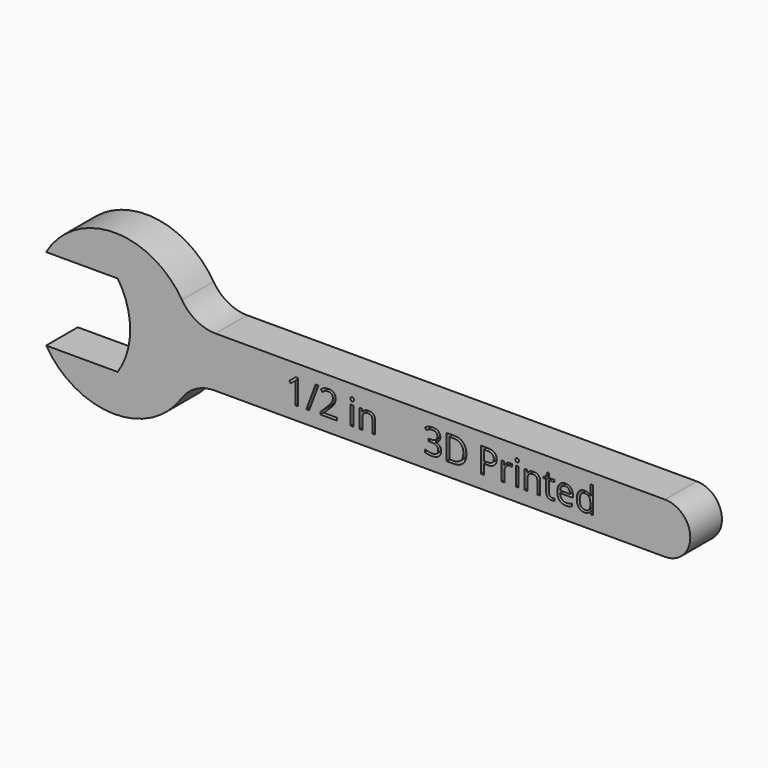
from build123d import *

# Parameters (mm, degrees)
F1_DEPTH     = 6.35
F2_TEXT_SIZE = 5.5941565531
F3_DEPTH     = 2


# Not quite as in the source:
# - Text() gives the source's letters only with a copy of the font that has no kerning and outlines rounded to 1/6400 em; it was checked with that copy


with BuildPart() as f1:
    # F0 (on Front) → F1 (new body)
    with BuildSketch(Plane.XZ):
        with BuildLine():
            Line((53.5489660396, 8.1024769281), (-18.6246478565, 8.1024769281))
            ThreePointArc((-18.6246478565, 8.1024769281), (-21.707286584, 8.900915123), (-24.0147138151, 11.0954411877))
            ThreePointArc((-24.0147138151, 11.0954411877), (-35.014283693, 17.0959234193), (-45.8292585891, 10.7687880083))
            Line((-45.8292585891, 10.7687880083), (-34.3312044384, 10.7687880083))
            ThreePointArc((-34.3312044384, 10.7687880083), (-32.3274172275, 4.1647880083), (-34.3312044384, -2.4392119917))
            Line((-34.3312044384, -2.4392119917), (-45.8206947839, -2.4392119917))
            ThreePointArc((-45.8206947839, -2.4392119917), (-35.0509770881, -8.5655910788), (-24.0725254588, -2.8216429775))
            ThreePointArc((-24.0725254588, -2.8216429775), (-21.7861297168, -0.7496621936), (-18.7930182164, 0))
            Line((-18.7930182164, 0), (53.5489660396, 0))
            Line((53.5489660396, 0), (53.5489660396, 8.1024769281))
        make_face()
        with BuildLine():
            ThreePointArc((53.5489660396, 0), (57.6002045036, 4.051238464), (53.5489660396, 8.1024769281))
            Line((53.5489660396, 8.1024769281), (53.5489660396, 0))
        make_face()
    extrude(amount=F1_DEPTH)

    # F2 (on face) → F3 (cut)
    with BuildSketch(Plane.XZ.offset(6.35)):
        with Locations((-7.3003843427, 2.1257819608)):
            Text('1/2 in     3D Printed', F2_TEXT_SIZE, font='Open Sans', text_align=(TextAlign.LEFT, TextAlign.BOTTOM))
    extrude(amount=-F3_DEPTH, mode=Mode.SUBTRACT)


solid = f1.part
